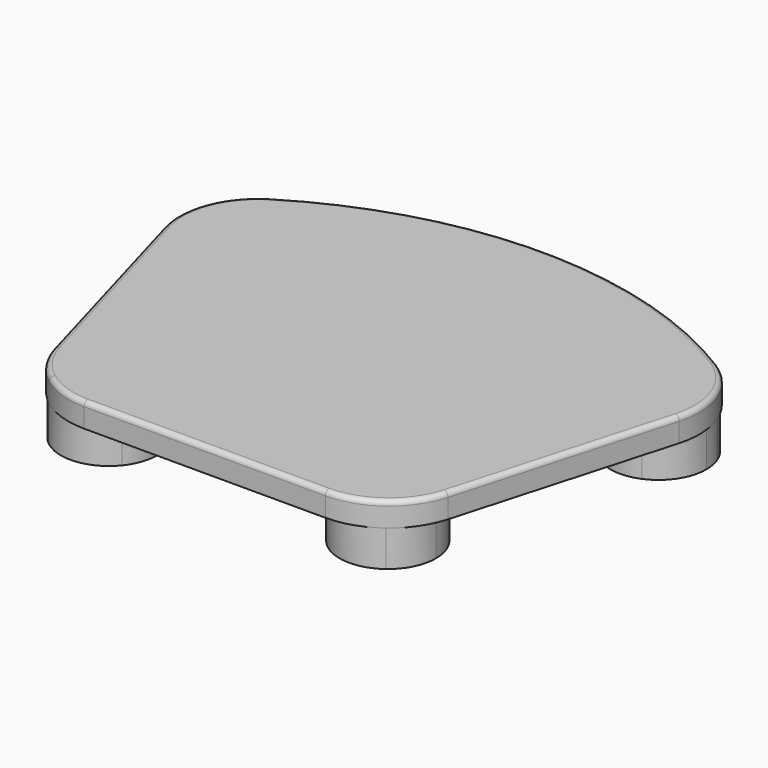
from build123d import *

# Parameters (mm, degrees)
F0_R     = 15
F1_DEPTH = 5
F2_DEPTH = 25
F3_DEPTH = 10
F4_R     = 2
F5_R     = 4.99999


# Not quite as in the source:
# - a fillet or chamfer is up to 0.001 mm smaller than in the source, because OpenCascade refuses the exact size


with BuildPart() as f1:
    # F0 (on Top) → F1 (new body)
    with BuildSketch(Plane.XY):
        with BuildLine():
            ThreePointArc((-69.9604572753, 6.6701451311), (-60.5580982639, 1.7119414898), (-50.0672739559, 0))
            Line((-50.0672739559, 0), (0, 0))
            Line((0, 0), (50.0672739559, 0))
            ThreePointArc((50.0672739559, 0), (60.5580981143, 1.7119414396), (69.9604570235, 6.6701449408))
            ThreePointArc((69.9604570235, 6.6701449408), (55.5054965809, 2.7719722055), (42.3945375666, 10))
            Line((42.3945375666, 10), (0, 10))
            Line((0, 10), (-42.3945375666, 10))
            ThreePointArc((-42.3945375666, 10), (-55.5054967376, 2.7719721865), (-69.9604572753, 6.6701451311))
        make_face()
        with BuildLine():
            ThreePointArc((-81.8117970817, 23.9841666211), (-77.2988184727, 14.3601774893), (-69.9604572753, 6.6701451311))
            ThreePointArc((-69.9604572753, 6.6701451311), (-77.6595229381, 19.5101618836), (-74.2884904631, 34.0970663646))
            Line((-74.2884904631, 34.0970663646), (-95.2609399047, 107.9405346638))
            ThreePointArc((-95.2609399047, 107.9405346638), (-105.7969677746, 118.575139565), (-105.9999990268, 133.5438229737))
            ThreePointArc((-105.9999990268, 133.5438229737), (-108.1976112364, 123.1486082025), (-106.9780364185, 112.5938639221))
            Line((-106.9780364185, 112.5938639221), (-81.8117970817, 23.9841666211))
        make_face()
        with BuildLine():
            ThreePointArc((-74.2884904631, 34.0970663646), (-77.6595229381, 19.5101618836), (-69.9604572753, 6.6701451311))
            ThreePointArc((-69.9604572753, 6.6701451311), (-55.5054967376, 2.7719721865), (-42.3945375666, 10))
            Line((-42.3945375666, 10), (-49.8081265441, 10))
            ThreePointArc((-49.8081265441, 10), (-66.9463387327, 10.6595171883), (-72.2630455249, 26.9655255543))
            Line((-72.2630455249, 26.9655255543), (-74.2884904631, 34.0970663646))
        make_face()
        with BuildLine():
            ThreePointArc((-37.9039826023, 22.6276329803), (-51.8910863458, 41.7023565329), (-74.2884904631, 34.0970663646))
            Line((-74.2884904631, 34.0970663646), (-72.2630455249, 26.9655255543))
            ThreePointArc((-72.2630455249, 26.9655255543), (-55.7114890264, 37.4665336107), (-42.9039826023, 22.6276329803))
            ThreePointArc((-42.9039826023, 22.6276329803), (-44.7427166891, 15.4317258406), (-49.8081265441, 10))
            Line((-49.8081265441, 10), (-42.3945375666, 10))
            ThreePointArc((-42.3945375666, 10), (-39.0600326353, 15.9264726596), (-37.9039826023, 22.6276329803))
        make_face()
        with BuildLine():
            Line((-95.2609399047, 107.9405346638), (-74.2884904631, 34.0970663646))
            ThreePointArc((-74.2884904631, 34.0970663646), (-51.8910863458, 41.7023565329), (-37.9039826023, 22.6276329803))
            ThreePointArc((-37.9039826023, 22.6276329803), (-39.0600326353, 15.9264726596), (-42.3945375666, 10))
            Line((-42.3945375666, 10), (0, 10))
            Line((0, 10), (42.3945375666, 10))
            ThreePointArc((42.3945375666, 10), (45.8475077617, 38.5851207029), (74.2884904631, 34.0970663646))
            Line((74.2884904631, 34.0970663646), (95.2609399047, 107.9405346638))
            ThreePointArc((95.2609399047, 107.9405346638), (68.7504432386, 118.9679329691), (80.581606816, 145.1296132529))
            ThreePointArc((80.581606816, 145.1296132529), (0, 166), (-80.581606816, 145.1296132529))
            ThreePointArc((-80.581606816, 145.1296132529), (-70.991481481, 137.8123064736), (-67.3536444198, 126.3110185474))
            ThreePointArc((-67.3536444198, 126.3110185474), (-76.3569610493, 109.6055417553), (-95.2609399047, 107.9405346638))
        make_face()
        with BuildLine():
            ThreePointArc((77.9039826023, 22.6276329803), (75.8083045445, 13.7149871449), (69.9604570235, 6.6701449408))
            ThreePointArc((69.9604570235, 6.6701449408), (77.2988183836, 14.3601773591), (81.8117970817, 23.9841666211))
            Line((81.8117970817, 23.9841666211), (106.9780364185, 112.5938639221))
            ThreePointArc((106.9780364185, 112.5938639221), (108.1976112852, 123.1486071561), (105.9999997845, 133.5438210204))
            ThreePointArc((105.9999997845, 133.5438210204), (107.0123207142, 129.990209539), (107.3536444198, 126.3110185474))
            ThreePointArc((107.3536444198, 126.3110185474), (104.0591212119, 115.3143351769), (95.2609399047, 107.9405346638))
            Line((95.2609399047, 107.9405346638), (74.2884904631, 34.0970663646))
            ThreePointArc((74.2884904631, 34.0970663646), (76.9787061549, 28.6405292368), (77.9039826023, 22.6276329803))
        make_face()
        with BuildLine():
            ThreePointArc((42.3945375666, 10), (55.5054965809, 2.7719722055), (69.9604570235, 6.6701449408))
            ThreePointArc((69.9604570235, 6.6701449408), (75.8083045445, 13.7149871449), (77.9039826023, 22.6276329803))
            ThreePointArc((77.9039826023, 22.6276329803), (76.9787061549, 28.6405292368), (74.2884904631, 34.0970663646))
            Line((74.2884904631, 34.0970663646), (72.2630455249, 26.9655255543))
            ThreePointArc((72.2630455249, 26.9655255543), (72.7428832327, 24.8201265562), (72.9039826023, 22.6276329803))
            ThreePointArc((72.9039826023, 22.6276329803), (65.099889742, 9.4663670672), (49.8081265441, 10))
            Line((49.8081265441, 10), (42.3945375666, 10))
        make_face()
        with BuildLine():
            ThreePointArc((-42.9039826023, 22.6276329803), (-55.7114890264, 37.4665336107), (-72.2630455249, 26.9655255543))
            Line((-72.2630455249, 26.9655255543), (-72.1922446193, 26.716237342))
            ThreePointArc((-72.1922446193, 26.716237342), (-63.9322200226, 14.648889119), (-50.0672739559, 10))
            Line((-50.0672739559, 10), (-49.8081265441, 10))
            ThreePointArc((-49.8081265441, 10), (-44.7427166891, 15.4317258406), (-42.9039826023, 22.6276329803))
        make_face()
        with BuildLine():
            Line((-72.1922446193, 26.716237342), (-72.2630455249, 26.9655255543))
            ThreePointArc((-72.2630455249, 26.9655255543), (-66.9463387327, 10.6595171883), (-49.8081265441, 10))
            Line((-49.8081265441, 10), (-50.0672739559, 10))
            ThreePointArc((-50.0672739559, 10), (-63.9322200226, 14.648889119), (-72.1922446193, 26.716237342))
        make_face()
        with BuildLine():
            ThreePointArc((-105.9999990268, 133.5438229737), (-105.7969677746, 118.575139565), (-95.2609399047, 107.9405346638))
            ThreePointArc((-95.2609399047, 107.9405346638), (-76.3569610493, 109.6055417553), (-67.3536444198, 126.3110185474))
            ThreePointArc((-67.3536444198, 126.3110185474), (-70.991481481, 137.8123064736), (-80.581606816, 145.1296132529))
            ThreePointArc((-80.581606816, 145.1296132529), (-95.6486721577, 144.5097139629), (-105.9999990268, 133.5438229737))
        make_face()
        with Locations((-87.3536444198, 126.3110185474)):
            Circle(F0_R, mode=Mode.SUBTRACT)
        with BuildLine():
            ThreePointArc((74.2884904631, 34.0970663646), (45.8475077617, 38.5851207029), (42.3945375666, 10))
            Line((42.3945375666, 10), (49.8081265441, 10))
            ThreePointArc((49.8081265441, 10), (48.8616264718, 34.5957487723), (72.2630455249, 26.9655255543))
            Line((72.2630455249, 26.9655255543), (74.2884904631, 34.0970663646))
        make_face()
        with BuildLine():
            ThreePointArc((-92.5950932834, 149.6734736012), (-100.6130145672, 142.701897638), (-105.9999990268, 133.5438229737))
            ThreePointArc((-105.9999990268, 133.5438229737), (-95.6486721577, 144.5097139629), (-80.581606816, 145.1296132529))
            ThreePointArc((-80.581606816, 145.1296132529), (0, 166), (80.581606816, 145.1296132529))
            ThreePointArc((80.581606816, 145.1296132529), (95.6486731109, 144.5097135284), (105.9999997845, 133.5438210204))
            ThreePointArc((105.9999997845, 133.5438210204), (100.6130152368, 142.7018968323), (92.5950932834, 149.6734736012))
            ThreePointArc((92.5950932834, 149.6734736012), (0, 176), (-92.5950932834, 149.6734736012))
        make_face()
        with BuildLine():
            ThreePointArc((72.2630455249, 26.9655255543), (48.8616264718, 34.5957487723), (49.8081265441, 10))
            Line((49.8081265441, 10), (50.0672739559, 10))
            ThreePointArc((50.0672739559, 10), (63.9322200226, 14.648889119), (72.1922446193, 26.716237342))
            Line((72.1922446193, 26.716237342), (72.2630455249, 26.9655255543))
        make_face()
        with BuildLine():
            Line((50.0672739559, 10), (49.8081265441, 10))
            ThreePointArc((49.8081265441, 10), (65.099889742, 9.4663670672), (72.9039826023, 22.6276329803))
            ThreePointArc((72.9039826023, 22.6276329803), (72.7428832327, 24.8201265562), (72.2630455249, 26.9655255543))
            Line((72.2630455249, 26.9655255543), (72.1922446193, 26.716237342))
            ThreePointArc((72.1922446193, 26.716237342), (63.9322200226, 14.648889119), (50.0672739559, 10))
        make_face()
        with BuildLine():
            ThreePointArc((107.3536444198, 126.3110185474), (107.0123207142, 129.990209539), (105.9999997845, 133.5438210204))
            ThreePointArc((105.9999997845, 133.5438210204), (95.6486731109, 144.5097135284), (80.581606816, 145.1296132529))
            ThreePointArc((80.581606816, 145.1296132529), (68.7504432386, 118.9679329691), (95.2609399047, 107.9405346638))
            ThreePointArc((95.2609399047, 107.9405346638), (104.0591212119, 115.3143351769), (107.3536444198, 126.3110185474))
        make_face()
        with Locations((87.3536444198, 126.3110185474)):
            Circle(F0_R, mode=Mode.SUBTRACT)
        with Locations((-87.3536444198, 126.3110185474)):
            Circle(F0_R)
        with Locations((87.3536444198, 126.3110185474)):
            Circle(F0_R)
    extrude(amount=-F1_DEPTH)

    # F0 (on Top) → F2 (join)
    with BuildSketch(Plane.XY):
        with BuildLine():
            ThreePointArc((-74.2884904631, 34.0970663646), (-77.6595229381, 19.5101618836), (-69.9604572753, 6.6701451311))
            ThreePointArc((-69.9604572753, 6.6701451311), (-55.5054967376, 2.7719721865), (-42.3945375666, 10))
            Line((-42.3945375666, 10), (-49.8081265441, 10))
            ThreePointArc((-49.8081265441, 10), (-66.9463387327, 10.6595171883), (-72.2630455249, 26.9655255543))
            Line((-72.2630455249, 26.9655255543), (-74.2884904631, 34.0970663646))
        make_face()
        with BuildLine():
            ThreePointArc((-37.9039826023, 22.6276329803), (-51.8910863458, 41.7023565329), (-74.2884904631, 34.0970663646))
            Line((-74.2884904631, 34.0970663646), (-72.2630455249, 26.9655255543))
            ThreePointArc((-72.2630455249, 26.9655255543), (-55.7114890264, 37.4665336107), (-42.9039826023, 22.6276329803))
            ThreePointArc((-42.9039826023, 22.6276329803), (-44.7427166891, 15.4317258406), (-49.8081265441, 10))
            Line((-49.8081265441, 10), (-42.3945375666, 10))
            ThreePointArc((-42.3945375666, 10), (-39.0600326353, 15.9264726596), (-37.9039826023, 22.6276329803))
        make_face()
        with BuildLine():
            ThreePointArc((42.3945375666, 10), (55.5054965809, 2.7719722055), (69.9604570235, 6.6701449408))
            ThreePointArc((69.9604570235, 6.6701449408), (75.8083045445, 13.7149871449), (77.9039826023, 22.6276329803))
            ThreePointArc((77.9039826023, 22.6276329803), (76.9787061549, 28.6405292368), (74.2884904631, 34.0970663646))
            Line((74.2884904631, 34.0970663646), (72.2630455249, 26.9655255543))
            ThreePointArc((72.2630455249, 26.9655255543), (72.7428832327, 24.8201265562), (72.9039826023, 22.6276329803))
            ThreePointArc((72.9039826023, 22.6276329803), (65.099889742, 9.4663670672), (49.8081265441, 10))
            Line((49.8081265441, 10), (42.3945375666, 10))
        make_face()
        with BuildLine():
            ThreePointArc((-105.9999990268, 133.5438229737), (-105.7969677746, 118.575139565), (-95.2609399047, 107.9405346638))
            ThreePointArc((-95.2609399047, 107.9405346638), (-76.3569610493, 109.6055417553), (-67.3536444198, 126.3110185474))
            ThreePointArc((-67.3536444198, 126.3110185474), (-70.991481481, 137.8123064736), (-80.581606816, 145.1296132529))
            ThreePointArc((-80.581606816, 145.1296132529), (-95.6486721577, 144.5097139629), (-105.9999990268, 133.5438229737))
        make_face()
        with Locations((-87.3536444198, 126.3110185474)):
            Circle(F0_R, mode=Mode.SUBTRACT)
        with BuildLine():
            ThreePointArc((74.2884904631, 34.0970663646), (45.8475077617, 38.5851207029), (42.3945375666, 10))
            Line((42.3945375666, 10), (49.8081265441, 10))
            ThreePointArc((49.8081265441, 10), (48.8616264718, 34.5957487723), (72.2630455249, 26.9655255543))
            Line((72.2630455249, 26.9655255543), (74.2884904631, 34.0970663646))
        make_face()
        with BuildLine():
            ThreePointArc((107.3536444198, 126.3110185474), (107.0123207142, 129.990209539), (105.9999997845, 133.5438210204))
            ThreePointArc((105.9999997845, 133.5438210204), (95.6486731109, 144.5097135284), (80.581606816, 145.1296132529))
            ThreePointArc((80.581606816, 145.1296132529), (68.7504432386, 118.9679329691), (95.2609399047, 107.9405346638))
            ThreePointArc((95.2609399047, 107.9405346638), (104.0591212119, 115.3143351769), (107.3536444198, 126.3110185474))
        make_face()
        with Locations((87.3536444198, 126.3110185474)):
            Circle(F0_R, mode=Mode.SUBTRACT)
    extrude(amount=-F2_DEPTH)

    # F0 (on Top) → F3 (join)
    with BuildSketch(Plane.XY):
        with BuildLine():
            ThreePointArc((-69.9604572753, 6.6701451311), (-60.5580982639, 1.7119414898), (-50.0672739559, 0))
            Line((-50.0672739559, 0), (0, 0))
            Line((0, 0), (50.0672739559, 0))
            ThreePointArc((50.0672739559, 0), (60.5580981143, 1.7119414396), (69.9604570235, 6.6701449408))
            ThreePointArc((69.9604570235, 6.6701449408), (55.5054965809, 2.7719722055), (42.3945375666, 10))
            Line((42.3945375666, 10), (0, 10))
            Line((0, 10), (-42.3945375666, 10))
            ThreePointArc((-42.3945375666, 10), (-55.5054967376, 2.7719721865), (-69.9604572753, 6.6701451311))
        make_face()
        with BuildLine():
            ThreePointArc((-81.8117970817, 23.9841666211), (-77.2988184727, 14.3601774893), (-69.9604572753, 6.6701451311))
            ThreePointArc((-69.9604572753, 6.6701451311), (-77.6595229381, 19.5101618836), (-74.2884904631, 34.0970663646))
            Line((-74.2884904631, 34.0970663646), (-95.2609399047, 107.9405346638))
            ThreePointArc((-95.2609399047, 107.9405346638), (-105.7969677746, 118.575139565), (-105.9999990268, 133.5438229737))
            ThreePointArc((-105.9999990268, 133.5438229737), (-108.1976112364, 123.1486082025), (-106.9780364185, 112.5938639221))
            Line((-106.9780364185, 112.5938639221), (-81.8117970817, 23.9841666211))
        make_face()
        with BuildLine():
            ThreePointArc((-92.5950932834, 149.6734736012), (-100.6130145672, 142.701897638), (-105.9999990268, 133.5438229737))
            ThreePointArc((-105.9999990268, 133.5438229737), (-95.6486721577, 144.5097139629), (-80.581606816, 145.1296132529))
            ThreePointArc((-80.581606816, 145.1296132529), (0, 166), (80.581606816, 145.1296132529))
            ThreePointArc((80.581606816, 145.1296132529), (95.6486731109, 144.5097135284), (105.9999997845, 133.5438210204))
            ThreePointArc((105.9999997845, 133.5438210204), (100.6130152368, 142.7018968323), (92.5950932834, 149.6734736012))
            ThreePointArc((92.5950932834, 149.6734736012), (0, 176), (-92.5950932834, 149.6734736012))
        make_face()
        with BuildLine():
            ThreePointArc((77.9039826023, 22.6276329803), (75.8083045445, 13.7149871449), (69.9604570235, 6.6701449408))
            ThreePointArc((69.9604570235, 6.6701449408), (77.2988183836, 14.3601773591), (81.8117970817, 23.9841666211))
            Line((81.8117970817, 23.9841666211), (106.9780364185, 112.5938639221))
            ThreePointArc((106.9780364185, 112.5938639221), (108.1976112852, 123.1486071561), (105.9999997845, 133.5438210204))
            ThreePointArc((105.9999997845, 133.5438210204), (107.0123207142, 129.990209539), (107.3536444198, 126.3110185474))
            ThreePointArc((107.3536444198, 126.3110185474), (104.0591212119, 115.3143351769), (95.2609399047, 107.9405346638))
            Line((95.2609399047, 107.9405346638), (74.2884904631, 34.0970663646))
            ThreePointArc((74.2884904631, 34.0970663646), (76.9787061549, 28.6405292368), (77.9039826023, 22.6276329803))
        make_face()
    extrude(amount=-F3_DEPTH)

    # F4
    f4_edges = [f1.edges().sort_by_distance(p)[0] for p in [
        (94.394917, 68.289015, 0),
        (106, 133.54382, 0),
        (0, 176, 0),
        (-106, 133.54382, 0),
        (-94.394917, 68.289015, 0),
        (-69.960457, 6.670145, 0),
        (0, 0, 0),
        (69.960457, 6.670145, 0),
        (-43.54492, 18.28974, -25),
        (65.999839, 35.255266, -25),
        (72.353644, 126.311019, -25),
        (-102.353644, 126.311019, -25),
    ]]
    fillet(f4_edges, radius=F4_R)

    # F5 (radius 5 in the source; OpenCascade refuses exactly that, so slightly less here)
    f5_edges = [f1.edges().sort_by_distance(p)[0] for p in [
        (45.847508, 38.585121, -5),
        (0, 10, -5),
        (-45.847508, 38.585121, -5),
        (-84.774715, 71.018801, -5),
        (-68.750443, 118.967933, -5),
        (0, 166, -5),
        (68.750443, 118.967933, -5),
        (84.774715, 71.018801, -5),
    ]]
    fillet(f5_edges, radius=F5_R)


solid = f1.part
